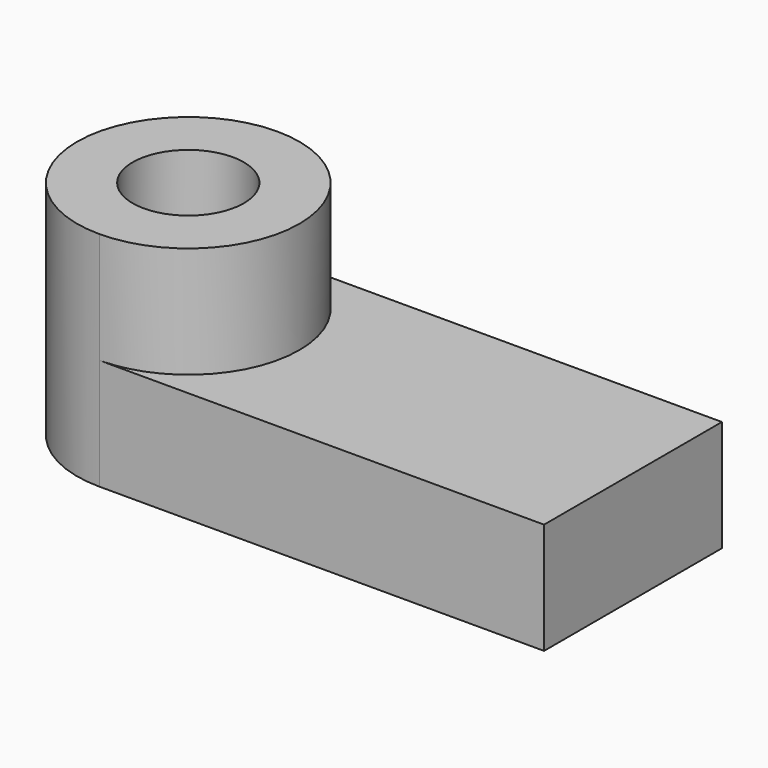
from build123d import *

# Parameters (mm, degrees)
F0_R     = 10
F1_DEPTH = 40
F2_DEPTH = 20


# Not quite as in the source:
# - ends of sketch curves that miss each other by under 0.0002 mm in the source are joined


with BuildPart() as f1:
    # F0 (on Top) → F1 (new body)
    with BuildSketch(Plane.XY):
        with BuildLine():
            ThreePointArc((-108.6277332274, -19.9999968788), (-94.4928212548, -14.1381846275), (-88.6389067712, 0))
            ThreePointArc((-88.6389067712, 0), (-94.4928212535, 14.1381846263), (-108.6277332239, 19.9999968788))
            ThreePointArc((-108.6277332239, 19.9999968788), (-128.6389067712, 1.7e-09), (-108.6277332274, -19.9999968788))
        make_face()
        with Locations((-108.6389067712, 0)):
            Circle(F0_R, mode=Mode.SUBTRACT)
    extrude(amount=F1_DEPTH)

    # F0 (on Top) → F2 (join)
    with BuildSketch(Plane.XY):
        with BuildLine():
            ThreePointArc((-108.6277332239, 19.9999968788), (-94.4928212535, 14.1381846263), (-88.6389067712, 0))
            ThreePointArc((-88.6389067712, 0), (-94.4928212548, -14.1381846275), (-108.6277332274, -19.9999968788))
            Line((-108.6277332274, -19.9999968788), (-28.6277332239, -20.0000031212))
            Line((-28.6277332239, -20.0000031212), (-28.6277332239, 19.9999968788))
            Line((-28.6277332239, 19.9999968788), (-108.6277332239, 19.9999968788))
        make_face()
    extrude(amount=F2_DEPTH)


solid = f1.part
